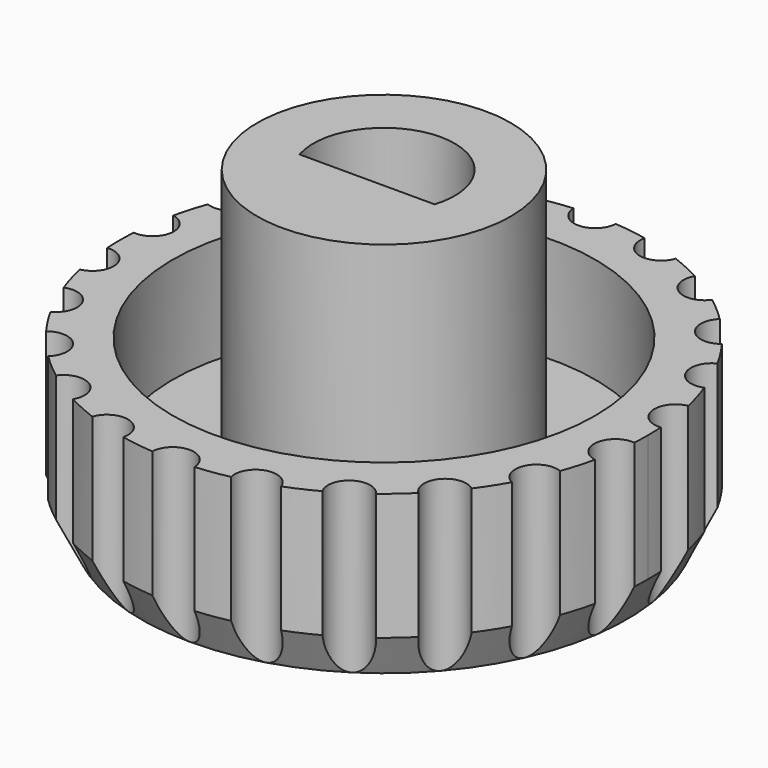
from build123d import *

# Parameters (mm, degrees)
F1_DEPTH = 8
F0_R     = 6
F2_DEPTH = 3
F3_DEPTH = 15
F4_DEPTH = 6
F7_DEPTH = 0.5
F8_R     = 0.49999


# Not quite as in the source:
# - a fillet or chamfer is up to 0.001 mm smaller than in the source, because OpenCascade refuses the exact size


with BuildPart() as f1:
    # F0 (on Top) → F1 (new body)
    with BuildSketch(Plane.XY):
        with BuildLine():
            ThreePointArc((12.4753761067, -0.7842136172), (12.4938425101, -0.3923000553), (12.5, 0))
            ThreePointArc((12.5, 0), (12.4938425101, 0.3923000553), (12.4753761067, 0.7842136172))
            ThreePointArc((12.4753761067, 0.7842136172), (11.3829465816, 1.6366206401), (12.190974225, 2.7622721526))
            ThreePointArc((12.190974225, 2.7622721526), (11.9936621702, 3.5216569605), (11.7490972101, 4.2671670636))
            ThreePointArc((11.7490972101, 4.2671670636), (10.4607679466, 4.7772726495), (10.9189321142, 6.0849750604))
            ThreePointArc((10.9189321142, 6.0849750604), (10.5156691604, 6.7580102182), (10.0709763321, 7.4044200123))
            ThreePointArc((10.0709763321, 7.4044200123), (8.6911201051, 7.5308984404), (8.7623030608, 8.9147094776))
            ThreePointArc((8.7623030608, 8.9147094776), (8.1857591743, 9.4468696794), (7.5769648461, 9.9418108874))
            ThreePointArc((7.5769648461, 9.9418108874), (6.2173694007, 9.6744156276), (5.8958043249, 11.0222271507))
            ThreePointArc((5.8958043249, 11.0222271507), (5.1926876625, 11.3703999419), (4.4691127302, 11.6737753707))
            ThreePointArc((4.4691127302, 11.6737753707), (3.2399244037, 11.0341691966), (2.5516625863, 12.2367895318))
            ThreePointArc((2.5516625863, 12.2367895318), (1.7789354784, 12.3727680235), (0.9991996797, 12.46))
            ThreePointArc((0.9991996797, 12.46), (0, 11.5), (-0.9991996797, 12.46))
            ThreePointArc((-0.9991996797, 12.46), (-1.7789354784, 12.3727680235), (-2.5516625863, 12.2367895318))
            ThreePointArc((-2.5516625863, 12.2367895318), (-3.2399244037, 11.0341691966), (-4.4691127302, 11.6737753707))
            ThreePointArc((-4.4691127302, 11.6737753707), (-5.1926876625, 11.3703999419), (-5.8958043249, 11.0222271507))
            ThreePointArc((-5.8958043249, 11.0222271507), (-6.2173694007, 9.6744156276), (-7.5769648461, 9.9418108874))
            ThreePointArc((-7.5769648461, 9.9418108874), (-8.1857591743, 9.4468696794), (-8.7623030608, 8.9147094776))
            ThreePointArc((-8.7623030608, 8.9147094776), (-8.6911201051, 7.5308984404), (-10.0709763321, 7.4044200123))
            ThreePointArc((-10.0709763321, 7.4044200123), (-10.5156691604, 6.7580102182), (-10.9189321142, 6.0849750604))
            ThreePointArc((-10.9189321142, 6.0849750604), (-10.4607679466, 4.7772726495), (-11.7490972101, 4.2671670636))
            ThreePointArc((-11.7490972101, 4.2671670636), (-11.9936621702, 3.5216569605), (-12.190974225, 2.7622721526))
            ThreePointArc((-12.190974225, 2.7622721526), (-11.3829465816, 1.6366206401), (-12.4753761067, 0.7842136172))
            ThreePointArc((-12.4753761067, 0.7842136172), (-12.5, 0), (-12.4753761067, -0.7842136172))
            ThreePointArc((-12.4753761067, -0.7842136172), (-11.3829465816, -1.6366206401), (-12.190974225, -2.7622721526))
            ThreePointArc((-12.190974225, -2.7622721526), (-11.9936621702, -3.5216569605), (-11.7490972101, -4.2671670636))
            ThreePointArc((-11.7490972101, -4.2671670636), (-10.4607679466, -4.7772726495), (-10.9189321142, -6.0849750604))
            ThreePointArc((-10.9189321142, -6.0849750604), (-10.5156691604, -6.7580102182), (-10.0709763321, -7.4044200123))
            ThreePointArc((-10.0709763321, -7.4044200123), (-8.6911201051, -7.5308984404), (-8.7623030608, -8.9147094776))
            ThreePointArc((-8.7623030608, -8.9147094776), (-8.1857591743, -9.4468696794), (-7.5769648461, -9.9418108874))
            ThreePointArc((-7.5769648461, -9.9418108874), (-6.2173694007, -9.6744156276), (-5.8958043249, -11.0222271507))
            ThreePointArc((-5.8958043249, -11.0222271507), (-5.1926876625, -11.3703999419), (-4.4691127302, -11.6737753707))
            ThreePointArc((-4.4691127302, -11.6737753707), (-3.2399244037, -11.0341691966), (-2.5516625863, -12.2367895318))
            ThreePointArc((-2.5516625863, -12.2367895318), (-1.7789354784, -12.3727680235), (-0.9991996797, -12.46))
            ThreePointArc((-0.9991996797, -12.46), (0, -11.5), (0.9991996797, -12.46))
            ThreePointArc((0.9991996797, -12.46), (1.7789354784, -12.3727680235), (2.5516625863, -12.2367895318))
            ThreePointArc((2.5516625863, -12.2367895318), (3.2399244037, -11.0341691966), (4.4691127302, -11.6737753707))
            ThreePointArc((4.4691127302, -11.6737753707), (5.1926876625, -11.3703999419), (5.8958043249, -11.0222271507))
            ThreePointArc((5.8958043249, -11.0222271507), (6.2173694007, -9.6744156276), (7.5769648461, -9.9418108874))
            ThreePointArc((7.5769648461, -9.9418108874), (8.1857591743, -9.4468696794), (8.7623030608, -8.9147094776))
            ThreePointArc((8.7623030608, -8.9147094776), (8.6911201051, -7.5308984404), (10.0709763321, -7.4044200123))
            ThreePointArc((10.0709763321, -7.4044200123), (10.5156691604, -6.7580102182), (10.9189321142, -6.0849750604))
            ThreePointArc((10.9189321142, -6.0849750604), (10.4607679466, -4.7772726495), (11.7490972101, -4.2671670636))
            ThreePointArc((11.7490972101, -4.2671670636), (11.9936621702, -3.5216569605), (12.190974225, -2.7622721526))
            ThreePointArc((12.190974225, -2.7622721526), (11.3829465816, -1.6366206401), (12.4753761067, -0.7842136172))
        make_face()
        with BuildLine():
            ThreePointArc((8.3768125793, -5.4615941822), (-9.5856175021, 2.848848382), (10, 0))
            ThreePointArc((10, 0), (9.5856175021, -2.848848382), (8.3768125793, -5.4615941822))
        make_face(mode=Mode.SUBTRACT)
    extrude(amount=F1_DEPTH)

    # F0 (on Top) → F2 (join)
    with BuildSketch(Plane.XY):
        with BuildLine():
            ThreePointArc((8.3768125793, -5.4615941822), (9.5856175021, -2.848848382), (10, 0))
            ThreePointArc((10, 0), (-9.5856175021, 2.848848382), (8.3768125793, -5.4615941822))
        make_face()
        with BuildLine():
            ThreePointArc((8.457975, -5.1885097957), (8.4372550797, -5.330954891), (8.3768125793, -5.4615941822))
            ThreePointArc((8.3768125793, -5.4615941822), (7.4786949203, -5.0460647004), (8.457975, -5.1885097957))
        make_face(mode=Mode.SUBTRACT)
        Circle(F0_R, mode=Mode.SUBTRACT)
        with BuildLine():
            ThreePointArc((8.457975, -5.1885097957), (7.4786949203, -5.0460647004), (8.3768125793, -5.4615941822))
            ThreePointArc((8.3768125793, -5.4615941822), (8.4372550797, -5.330954891), (8.457975, -5.1885097957))
        make_face()
    extrude(amount=F2_DEPTH)

    # F0 (on Top) → F3 (join)
    with BuildSketch(Plane.XY):
        Circle(F0_R)
        with BuildLine():
            ThreePointArc((-3.1972644557, -1), (0, 3.35), (3.1972644557, -1))
            Line((3.1972644557, -1), (-3.1972644557, -1))
        make_face(mode=Mode.SUBTRACT)
    extrude(amount=F3_DEPTH)

    # F0 (on Top) → F4 (join)
    with BuildSketch(Plane.XY):
        with BuildLine():
            Line((-3.1972644557, -1), (3.1972644557, -1))
            ThreePointArc((3.1972644557, -1), (0, 3.35), (-3.1972644557, -1))
        make_face()
    extrude(amount=F4_DEPTH)

    # F6: sweep along a path in F0
    with BuildLine(Plane.XY) as f6_path:
        CenterArc((0, 0), 12.5, 0, 360)
    # F5 (on Front) → F6 (sweep, cut)
    with BuildSketch(Plane.XZ):
        Polygon((-12.5, 2), (-12.5, 0), (-11.5, 0), align=None)
    sweep(path=f6_path.line, mode=Mode.SUBTRACT)

    # F0 (on Top) → F7 (cut)
    with BuildSketch(Plane.XY):
        with BuildLine():
            ThreePointArc((8.457975, -5.1885097957), (7.4786949203, -5.0460647004), (8.3768125793, -5.4615941822))
            ThreePointArc((8.3768125793, -5.4615941822), (8.4372550797, -5.330954891), (8.457975, -5.1885097957))
        make_face()
    extrude(amount=F7_DEPTH, mode=Mode.SUBTRACT)

    # F8 (radius 0.5 in the source; OpenCascade refuses exactly that, so slightly less here)
    f8_edges = [f1.edges().sort_by_distance(p)[0] for p in [
        (7.539137, -4.915425, 0.5),
    ]]
    fillet(f8_edges, radius=F8_R)


solid = f1.part
